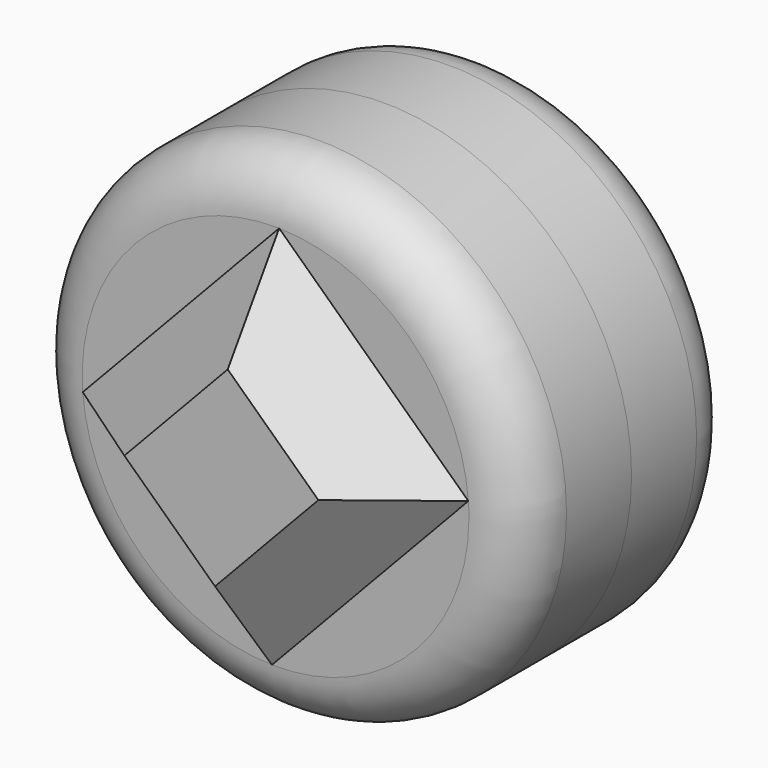
from build123d import *

# Parameters (mm, degrees)
F0_R     = 23.1993727041
F1_DEPTH = 12.7
F2_R     = 23.1993727041
F3_DEPTH = 12.7
F4_R     = 5.08
F7_DEPTH = 6.35
F8_DEPTH = 6.35
F9_SIZE  = 6.34999
F10_SIZE = 6.34999


# Not quite as in the source:
# - a fillet or chamfer is up to 0.001 mm smaller than in the source, because OpenCascade refuses the exact size


with BuildPart() as f1:
    # F0 (on Front) → F1 (new body)
    with BuildSketch(Plane.XZ):
        with Locations((-16.9251933694, -16.9251933694)):
            Circle(F0_R)
    extrude(amount=F1_DEPTH)

    # F2 (on face) → F3 (join)
    with BuildSketch(Plane(origin=(0, 0, 0), x_dir=(-1, 0, 0), z_dir=(0, 1, 0))):
        with Locations((16.9251933694, -16.9251933694)):
            Circle(F2_R)
    extrude(amount=F3_DEPTH)

    # F4
    f4_edges = [f1.edges().sort_by_distance(p)[0] for p in [
        (6.274179, 12.7, -16.925193),
        (-16.925193, 0, 6.274179),
        (-16.925193, 0, -40.124566),
        (6.274179, -6.35, -16.925193),
        (-40.124566, -12.7, -16.925193),
        (-40.124566, 6.35, -16.925193),
    ]]
    fillet(f4_edges, radius=F4_R)

    # F5 (on face) → F7 (join)
    with BuildSketch(Plane(origin=(0, 12.7, 0), x_dir=(-1, 0, 0), z_dir=(0, 1, 0))):
        Polygon((34.987336153, -18.3641740003), (16.5690030176, 1.1906780042), (-1.1369494142, -15.4862127385), (17.2813837212, -35.041064743), align=None)
    extrude(amount=F7_DEPTH)

    # F6 (on face) → F8 (join)
    with BuildSketch(Plane.XZ.offset(12.7)):
        Polygon((1.1413726115, -15.5428544637), (-16.5892601531, 1.1910649658), (-34.9917593503, -18.3075322751), (-17.2611265857, -35.0414517045), align=None)
    extrude(amount=F8_DEPTH)

    # F9 (size 6.35 in the source; OpenCascade refuses exactly that, so slightly less here)
    f9_edges = [f1.edges().sort_by_distance(p)[0] for p in [
        (-8.072217, 19.05, -25.263639),
        (-26.13436, 19.05, -26.702619),
        (-25.77817, 19.05, -8.586748),
        (-7.716027, 19.05, -7.147767),
    ]]
    chamfer(f9_edges, length=F9_SIZE)

    # F10 (size 6.35 in the source; OpenCascade refuses exactly that, so slightly less here)
    f10_edges = [f1.edges().sort_by_distance(p)[0] for p in [
        (-8.059877, -19.05, -25.292153),
        (-7.723944, -19.05, -7.175895),
        (-25.79051, -19.05, -8.558234),
        (-26.126443, -19.05, -26.674492),
    ]]
    chamfer(f10_edges, length=F10_SIZE)


solid = f1.part
